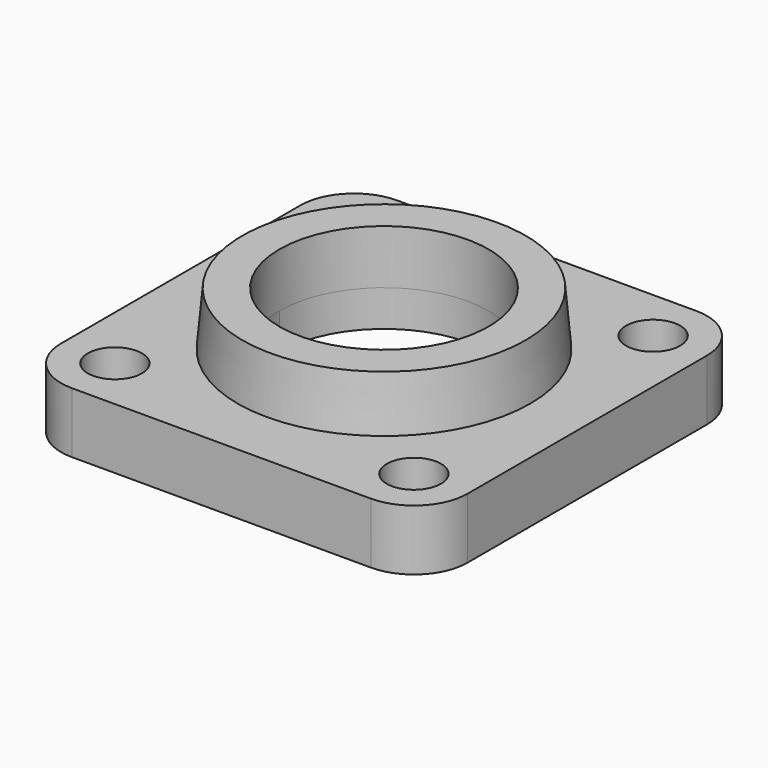
from build123d import *

# Parameters (mm, degrees)
F1_DEPTH        = 14.224
F2_DEPTH        = 5.715
F3_D            = 12.7
F3_COPIES_COUNT = 4
F5_R            = 34.29
F6_DEPTH        = 12.7
F6_TAPER        = 5
F7_D            = 49.022
F7_DEPTH        = 14.225
F8_D            = 49.022


# Not quite as in the source:
# - a pattern or mirror of a feature is missing from the dataset's text; its kind, count and spacing are read off the source's solid


with BuildPart() as f1:
    # F0 (on Top) → F1 (new body)
    with BuildSketch(Plane.XY):
        with BuildLine():
            Line((35.0229988722, 47.625), (-35.0229988722, 47.625))
            ThreePointArc((-35.0229988722, 47.625), (-43.9339593262, 43.9339593262), (-47.625, 35.0229988722))
            Line((-47.625, 35.0229988722), (-47.625, -35.0229988722))
            ThreePointArc((-47.625, -35.0229988722), (-43.9339593262, -43.9339593262), (-35.0229988722, -47.625))
            Line((-35.0229988722, -47.625), (35.0229988722, -47.625))
            ThreePointArc((35.0229988722, -47.625), (43.9339593262, -43.9339593262), (47.625, -35.0229988722))
            Line((47.625, -35.0229988722), (47.625, 35.0229988722))
            ThreePointArc((47.625, 35.0229988722), (43.9339593262, 43.9339593262), (35.0229988722, 47.625))
        make_face()
        with BuildLine():
            Line((22.3801912029, -40.005), (-22.3801912029, -40.005))
            ThreePointArc((-22.3801912029, -40.005), (-25.4141248226, -25.4141248226), (-40.005, -22.3801912029))
            Line((-40.005, -22.3801912029), (-40.005, 22.3801912029))
            ThreePointArc((-40.005, 22.3801912029), (-25.4141248226, 25.4141248226), (-22.3801912029, 40.005))
            Line((-22.3801912029, 40.005), (22.3801912029, 40.005))
            ThreePointArc((22.3801912029, 40.005), (25.4141248226, 25.4141248226), (40.005, 22.3801912029))
            Line((40.005, 22.3801912029), (40.005, -22.3801912029))
            ThreePointArc((40.005, -22.3801912029), (25.4141248226, -25.4141248226), (22.3801912029, -40.005))
        make_face(mode=Mode.SUBTRACT)
        with BuildLine():
            ThreePointArc((-40.005, -22.3801912029), (-25.4141248226, -25.4141248226), (-22.3801912029, -40.005))
            Line((-22.3801912029, -40.005), (22.3801912029, -40.005))
            ThreePointArc((22.3801912029, -40.005), (25.4141248226, -25.4141248226), (40.005, -22.3801912029))
            Line((40.005, -22.3801912029), (40.005, 22.3801912029))
            ThreePointArc((40.005, 22.3801912029), (25.4141248226, 25.4141248226), (22.3801912029, 40.005))
            Line((22.3801912029, 40.005), (-22.3801912029, 40.005))
            ThreePointArc((-22.3801912029, 40.005), (-25.4141248226, 25.4141248226), (-40.005, 22.3801912029))
            Line((-40.005, 22.3801912029), (-40.005, -22.3801912029))
        make_face()
    extrude(amount=F1_DEPTH)

    # F0 (on Top) → F2 (cut)
    with BuildSketch(Plane.XY):
        with BuildLine():
            ThreePointArc((-40.005, -22.3801912029), (-25.4141248226, -25.4141248226), (-22.3801912029, -40.005))
            Line((-22.3801912029, -40.005), (22.3801912029, -40.005))
            ThreePointArc((22.3801912029, -40.005), (25.4141248226, -25.4141248226), (40.005, -22.3801912029))
            Line((40.005, -22.3801912029), (40.005, 22.3801912029))
            ThreePointArc((40.005, 22.3801912029), (25.4141248226, 25.4141248226), (22.3801912029, 40.005))
            Line((22.3801912029, 40.005), (-22.3801912029, 40.005))
            ThreePointArc((-22.3801912029, 40.005), (-25.4141248226, 25.4141248226), (-40.005, 22.3801912029))
            Line((-40.005, 22.3801912029), (-40.005, -22.3801912029))
        make_face()
    extrude(amount=F2_DEPTH, mode=Mode.SUBTRACT)

    # F3 (through all)
    with Locations(Plane(origin=(0, 0, 0), x_dir=(1, 0, 0), z_dir=(0, 0, -1))):
        with Locations((-35.0229988722, -35.0229988722)):
            f3 = Hole(F3_D / 2)

    # F3_copies: F3 ×4 about axis
    f3_copies_axis = Axis((0, 0, 0), (0, 0, 1))
    for i in range(1, F3_COPIES_COUNT):
        add(f3.rotate(f3_copies_axis, i * 360 / F3_COPIES_COUNT), mode=Mode.SUBTRACT)

    # F5 (on face) → F6 (join)
    with BuildSketch(Plane.XY.offset(14.224)):
        Circle(F5_R)
    extrude(amount=F6_DEPTH, taper=F6_TAPER)

    # F7 (through all, one way)
    with BuildSketch(Plane.XY.offset(14.224)):
        with Locations((0, 0)):
            Circle(F7_D / 2)
    extrude(amount=-F7_DEPTH, mode=Mode.SUBTRACT)

    # F8 (through all)
    with Locations(Plane(origin=(0, 0, 14.224), x_dir=(1, 0, 0), z_dir=(0, 0, -1))):
        with Locations((0, 0)):
            Hole(F8_D / 2)


solid = f1.part
